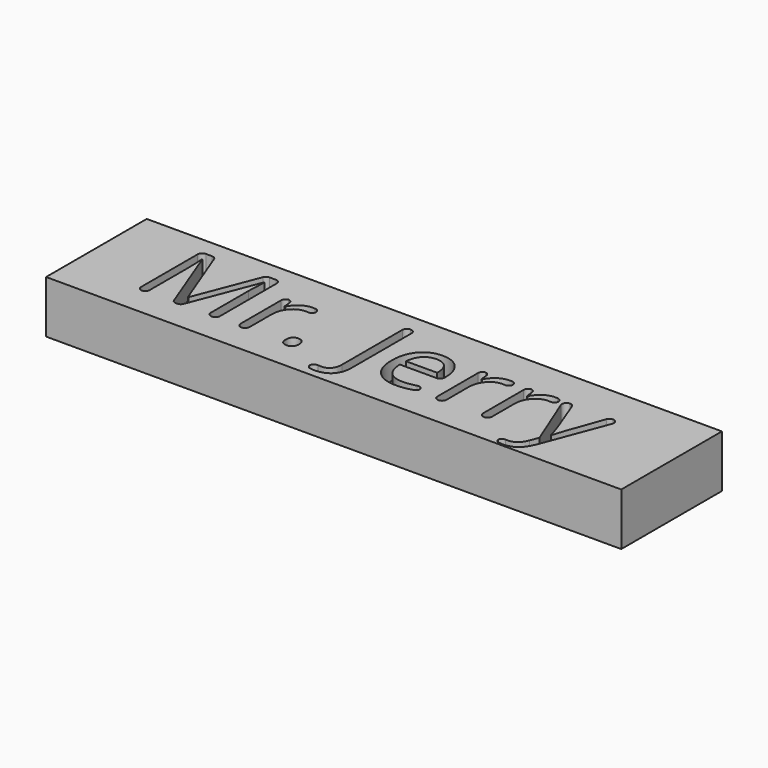
from build123d import *

# Parameters (mm, degrees)
F0_W         = 203.2
F0_H         = 44.45
F1_DEPTH     = 18.542
F2_TEXT_SIZE = 39.4664945685
F3_DEPTH     = 6.35
F4_T1_DEPTH  = 10.31875
F4_T3_DEPTH  = 9.0775000668
F4_T5_DEPTH  = 9.0694093583
F4_T7_DEPTH  = 9.9608913687
F4_T9_DEPTH  = 10.7046893029
F4_T11_DEPTH = 9.0805717525
F4_T13_DEPTH = 9.0709488545
F4_T15_DEPTH = 10.3720428243
F4_T17_DEPTH = 11.118182573
F4_T19_DEPTH = 9.8149761464
F4_T21_DEPTH = 9.1515288397
F4_T23_DEPTH = 11.9961106327
F4_T25_DEPTH = 9.0772375282
F4_T27_DEPTH = 9.1351619344
F4_T29_DEPTH = 12.2189306732
F4_T31_DEPTH = 12.0899797084
F4_T33_DEPTH = 10.8409697131
F4_T35_DEPTH = 9.9077155537


# Not quite as in the source:
# - a fillet or chamfer that OpenCascade refuses, or shapes differently, is made with other operations: its cross-section is extruded or revolved along the edge and cut away or added
# - Text() gives the source's letters only with a copy of the font that has no kerning and outlines rounded to 1/6400 em; it was checked with that copy


with BuildPart() as f1:
    # F0 (on Top) → F1 (new body)
    with BuildSketch(Plane.XY):
        with Locations((101.6, 22.225)):
            Rectangle(F0_W, F0_H)
    extrude(amount=F1_DEPTH)

    # F2 (on face) → F3 (cut)
    with BuildSketch(Plane.XY.offset(18.542)):
        with Locations((20.3022701502, 10.1437785078)):
            Text('Mr. Jerry', F2_TEXT_SIZE, font='Open Sans', text_align=(TextAlign.LEFT, TextAlign.BOTTOM))
    extrude(amount=-F3_DEPTH, mode=Mode.SUBTRACT)

    # F4: fillet of radius 1.5875 on 41 edges, made by hand

    # F4_s2 → F4_t1 (join)
    with BuildSketch(Plane.XY.offset(8.22325)):
        with BuildLine():
            ThreePointArc((25.7624199297, 38.3191556458), (24.6398879146, 37.8541876609), (24.1749199297, 36.7316556458))
            Line((24.1749199297, 36.7316556458), (24.1431699297, 36.7316556458))
            Line((24.1431699297, 36.7316556458), (24.1431699297, 38.3509056458))
            Line((24.1431699297, 38.3509056458), (25.7624199297, 38.3509056458))
            Line((25.7624199297, 38.3509056458), (25.7624199297, 38.3191556458))
        make_face()
        with BuildLine():
            ThreePointArc((52.0789649176, 36.7316556458), (51.6139969327, 37.8541876609), (50.4914649176, 38.3191556458))
            Line((50.4914649176, 38.3191556458), (50.4914649176, 38.3509056458))
            Line((50.4914649176, 38.3509056458), (52.1107149176, 38.3509056458))
            Line((52.1107149176, 38.3509056458), (52.1107149176, 36.7316556458))
            Line((52.1107149176, 36.7316556458), (52.0789649176, 36.7316556458))
        make_face()
        with BuildLine():
            ThreePointArc((60.9122666547, 31.2645197417), (59.7897346396, 30.7995517568), (59.3247666547, 29.6770197417))
            Line((59.3247666547, 29.6770197417), (59.2930166547, 29.6770197417))
            Line((59.2930166547, 29.6770197417), (59.2930166547, 31.2962697417))
            Line((59.2930166547, 31.2962697417), (60.9122666547, 31.2962697417))
            Line((60.9122666547, 31.2962697417), (60.9122666547, 31.2645197417))
        make_face()
        with BuildLine():
            ThreePointArc((25.6152400599, 10.1437785078), (26.737772075, 10.6087464926), (27.2027400599, 11.7312785078))
            Line((27.2027400599, 11.7312785078), (27.2344900599, 11.7312785078))
            Line((27.2344900599, 11.7312785078), (27.2344900599, 10.1120285078))
            Line((27.2344900599, 10.1120285078), (25.6152400599, 10.1120285078))
            Line((25.6152400599, 10.1120285078), (25.6152400599, 10.1437785078))
        make_face()
        with BuildLine():
            ThreePointArc((24.1749199297, 11.7312785078), (24.6398879146, 10.6087464926), (25.7624199297, 10.1437785078))
            Line((25.7624199297, 10.1437785078), (25.7624199297, 10.1120285078))
            Line((25.7624199297, 10.1120285078), (24.1431699297, 10.1120285078))
            Line((24.1431699297, 10.1120285078), (24.1431699297, 11.7312785078))
            Line((24.1431699297, 11.7312785078), (24.1749199297, 11.7312785078))
        make_face()
        with BuildLine():
            ThreePointArc((48.8044791963, 11.7312785078), (49.2694471812, 10.6087464926), (50.3919791963, 10.1437785078))
            Line((50.3919791963, 10.1437785078), (50.3919791963, 10.1120285078))
            Line((50.3919791963, 10.1120285078), (48.7727291963, 10.1120285078))
            Line((48.7727291963, 10.1120285078), (48.7727291963, 11.7312785078))
            Line((48.7727291963, 11.7312785078), (48.8044791963, 11.7312785078))
        make_face()
        with BuildLine():
            ThreePointArc((60.9377526987, 10.1437785078), (62.0602847138, 10.6087464926), (62.5252526987, 11.7312785078))
            Line((62.5252526987, 11.7312785078), (62.5570026987, 11.7312785078))
            Line((62.5570026987, 11.7312785078), (62.5570026987, 10.1120285078))
            Line((62.5570026987, 10.1120285078), (60.9377526987, 10.1120285078))
            Line((60.9377526987, 10.1120285078), (60.9377526987, 10.1437785078))
        make_face()
        with BuildLine():
            ThreePointArc((50.4914649176, 10.1437785078), (51.6139969327, 10.6087464926), (52.0789649176, 11.7312785078))
            Line((52.0789649176, 11.7312785078), (52.1107149176, 11.7312785078))
            Line((52.1107149176, 11.7312785078), (52.1107149176, 10.1120285078))
            Line((52.1107149176, 10.1120285078), (50.4914649176, 10.1120285078))
            Line((50.4914649176, 10.1120285078), (50.4914649176, 10.1437785078))
        make_face()
        with BuildLine():
            ThreePointArc((59.3247666547, 11.7312785078), (59.7897346396, 10.6087464926), (60.9122666547, 10.1437785078))
            Line((60.9122666547, 10.1437785078), (60.9122666547, 10.1120285078))
            Line((60.9122666547, 10.1120285078), (59.2930166547, 10.1120285078))
            Line((59.2930166547, 10.1120285078), (59.2930166547, 11.7312785078))
            Line((59.2930166547, 11.7312785078), (59.3247666547, 11.7312785078))
        make_face()
        with BuildLine():
            ThreePointArc((98.0539380275, 38.3191556458), (96.9314060124, 37.8541876609), (96.4664380275, 36.7316556458))
            Line((96.4664380275, 36.7316556458), (96.4346880275, 36.7316556458))
            Line((96.4346880275, 36.7316556458), (96.4346880275, 38.3509056458))
            Line((96.4346880275, 38.3509056458), (98.0539380275, 38.3509056458))
            Line((98.0539380275, 38.3509056458), (98.0539380275, 38.3191556458))
        make_face()
        with BuildLine():
            ThreePointArc((99.7409237488, 36.7316556458), (99.2759557639, 37.8541876609), (98.1534237488, 38.3191556458))
            Line((98.1534237488, 38.3191556458), (98.1534237488, 38.3509056458))
            Line((98.1534237488, 38.3509056458), (99.7726737488, 38.3509056458))
            Line((99.7726737488, 38.3509056458), (99.7726737488, 36.7316556458))
            Line((99.7726737488, 36.7316556458), (99.7409237488, 36.7316556458))
        make_face()
        with BuildLine():
            ThreePointArc((121.8333204898, 20.1275683056), (122.955852505, 20.5925362905), (123.4208204898, 21.7150683056))
            Line((123.4208204898, 21.7150683056), (123.4525704898, 21.7150683056))
            Line((123.4525704898, 21.7150683056), (123.4525704898, 20.0958183056))
            Line((123.4525704898, 20.0958183056), (121.8333204898, 20.0958183056))
            Line((121.8333204898, 20.0958183056), (121.8333204898, 20.1275683056))
        make_face()
        with BuildLine():
            ThreePointArc((130.4657966919, 31.2645197417), (129.3432646767, 30.7995517568), (128.8782966919, 29.6770197417))
            Line((128.8782966919, 29.6770197417), (128.8465466919, 29.6770197417))
            Line((128.8465466919, 29.6770197417), (128.8465466919, 31.2962697417))
            Line((128.8465466919, 31.2962697417), (130.4657966919, 31.2962697417))
            Line((130.4657966919, 31.2962697417), (130.4657966919, 31.2645197417))
        make_face()
        with BuildLine():
            ThreePointArc((128.8782966919, 11.7312785078), (129.3432646767, 10.6087464926), (130.4657966919, 10.1437785078))
            Line((130.4657966919, 10.1437785078), (130.4657966919, 10.1120285078))
            Line((130.4657966919, 10.1120285078), (128.8465466919, 10.1120285078))
            Line((128.8465466919, 10.1120285078), (128.8465466919, 11.7312785078))
            Line((128.8465466919, 11.7312785078), (128.8782966919, 11.7312785078))
        make_face()
        with BuildLine():
            ThreePointArc((130.4912827358, 10.1437785078), (131.6138147509, 10.6087464926), (132.0787827358, 11.7312785078))
            Line((132.0787827358, 11.7312785078), (132.1105327358, 11.7312785078))
            Line((132.1105327358, 11.7312785078), (132.1105327358, 10.1120285078))
            Line((132.1105327358, 10.1120285078), (130.4912827358, 10.1120285078))
            Line((130.4912827358, 10.1120285078), (130.4912827358, 10.1437785078))
        make_face()
        with BuildLine():
            ThreePointArc((146.5792264274, 31.2645197417), (145.4566944123, 30.7995517568), (144.9917264274, 29.6770197417))
            Line((144.9917264274, 29.6770197417), (144.9599764274, 29.6770197417))
            Line((144.9599764274, 29.6770197417), (144.9599764274, 31.2962697417))
            Line((144.9599764274, 31.2962697417), (146.5792264274, 31.2962697417))
            Line((146.5792264274, 31.2962697417), (146.5792264274, 31.2645197417))
        make_face()
        with BuildLine():
            ThreePointArc((144.9917264274, 11.7312785078), (145.4566944123, 10.6087464926), (146.5792264274, 10.1437785078))
            Line((146.5792264274, 10.1437785078), (146.5792264274, 10.1120285078))
            Line((146.5792264274, 10.1120285078), (144.9599764274, 10.1120285078))
            Line((144.9599764274, 10.1120285078), (144.9599764274, 11.7312785078))
            Line((144.9599764274, 11.7312785078), (144.9917264274, 11.7312785078))
        make_face()
        with BuildLine():
            ThreePointArc((146.6047124713, 10.1437785078), (147.7272444864, 10.6087464926), (148.1922124713, 11.7312785078))
            Line((148.1922124713, 11.7312785078), (148.2239624713, 11.7312785078))
            Line((148.2239624713, 11.7312785078), (148.2239624713, 10.1120285078))
            Line((148.2239624713, 10.1120285078), (146.6047124713, 10.1120285078))
            Line((146.6047124713, 10.1120285078), (146.6047124713, 10.1437785078))
        make_face()
    extrude(amount=F4_T1_DEPTH)

    # F4_s4 → F4_t3 (join)
    with BuildSketch(Plane.XY.offset(9.4644999332)):
        with BuildLine():
            ThreePointArc((29.4992621736, 37.3006389465), (28.9163688827, 38.0399784729), (28.0172317241, 38.3191556458))
            Line((28.0172317241, 38.3191556458), (28.0172317241, 38.3509056458))
            Line((28.0172317241, 38.3509056458), (29.1300517513, 38.3509056458))
            Line((29.1300517513, 38.3509056458), (29.5289027826, 37.3120186125))
            Line((29.5289027826, 37.3120186125), (29.4992621736, 37.3006389465))
        make_face()
    extrude(amount=F4_T3_DEPTH)

    # F4_s6 → F4_t5 (join)
    with BuildSketch(Plane.XY.offset(9.4725906417)):
        with BuildLine():
            ThreePointArc((48.2704166785, 38.3191556458), (47.3730936562, 38.0412233774), (46.7899690882, 37.3047448032))
            Line((46.7899690882, 37.3047448032), (46.7603601364, 37.3162065863))
            Line((46.7603601364, 37.3162065863), (47.1608976603, 38.3509056458))
            Line((47.1608976603, 38.3509056458), (48.2704166785, 38.3509056458))
            Line((48.2704166785, 38.3509056458), (48.2704166785, 38.3191556458))
        make_face()
    extrude(amount=F4_T5_DEPTH)

    # F4_s8 → F4_t7 (join)
    with BuildSketch(Plane.XY.offset(8.5811086313)):
        with BuildLine():
            ThreePointArc((62.100170343, 29.8265880456), (61.588075642, 30.8512420231), (60.5197319315, 31.2645197417))
            Line((60.5197319315, 31.2645197417), (60.5197319315, 31.2962697417))
            Line((60.5197319315, 31.2962697417), (61.99297561, 31.2962697417))
            Line((61.99297561, 31.2962697417), (62.1317791112, 29.8295794117))
            Line((62.1317791112, 29.8295794117), (62.100170343, 29.8265880456))
        make_face()
        with BuildLine():
            ThreePointArc((131.6537003801, 29.8265880456), (131.1416056791, 30.8512420231), (130.0732619686, 31.2645197417))
            Line((130.0732619686, 31.2645197417), (130.0732619686, 31.2962697417))
            Line((130.0732619686, 31.2962697417), (131.5465056471, 31.2962697417))
            Line((131.5465056471, 31.2962697417), (131.6853091483, 29.8295794117))
            Line((131.6853091483, 29.8295794117), (131.6537003801, 29.8265880456))
        make_face()
        with BuildLine():
            ThreePointArc((147.7671301156, 29.8265880456), (147.2550354147, 30.8512420231), (146.1866917042, 31.2645197417))
            Line((146.1866917042, 31.2645197417), (146.1866917042, 31.2962697417))
            Line((146.1866917042, 31.2962697417), (147.6599353826, 31.2962697417))
            Line((147.6599353826, 31.2962697417), (147.7987388839, 29.8295794117))
            Line((147.7987388839, 29.8295794117), (147.7671301156, 29.8265880456))
        make_face()
    extrude(amount=F4_T7_DEPTH)

    # F4_s10 → F4_t9 (join)
    with BuildSketch(Plane.XY.offset(7.8373106971)):
        with BuildLine():
            ThreePointArc((69.7567620656, 31.633185269), (70.9040374696, 31.0525772552), (71.2449954189, 29.8127812256))
            Line((71.2449954189, 29.8127812256), (71.2763955831, 29.8080809931))
            Line((71.2763955831, 29.8080809931), (71.5167804579, 31.4139855036))
            Line((71.5167804579, 31.4139855036), (71.4919038216, 31.4497583298))
            ThreePointArc((71.4919038216, 31.4497583298), (70.6289396634, 31.590880749), (69.7583975628, 31.6648931174))
            Line((69.7583975628, 31.6648931174), (69.7567620656, 31.633185269))
        make_face()
        with BuildLine():
            ThreePointArc((139.3102921027, 31.633185269), (140.4575675067, 31.0525772552), (140.798525456, 29.8127812256))
            Line((140.798525456, 29.8127812256), (140.8299256203, 29.8080809931))
            Line((140.8299256203, 29.8080809931), (141.070310495, 31.4139855036))
            Line((141.070310495, 31.4139855036), (141.0454338587, 31.4497583298))
            ThreePointArc((141.0454338587, 31.4497583298), (140.1824697005, 31.590880749), (139.3119275999, 31.6648931174))
            Line((139.3119275999, 31.6648931174), (139.3102921027, 31.633185269))
        make_face()
        with BuildLine():
            ThreePointArc((155.4237218383, 31.633185269), (156.5709972423, 31.0525772552), (156.9119551916, 29.8127812256))
            Line((156.9119551916, 29.8127812256), (156.9433553558, 29.8080809931))
            Line((156.9433553558, 29.8080809931), (157.1837402305, 31.4139855036))
            Line((157.1837402305, 31.4139855036), (157.1588635943, 31.4497583298))
            ThreePointArc((157.1588635943, 31.4497583298), (156.2958994361, 31.590880749), (155.4253573354, 31.6648931174))
            Line((155.4253573354, 31.6648931174), (155.4237218383, 31.633185269))
        make_face()
    extrude(amount=F4_T9_DEPTH)

    # F4_s12 → F4_t11 (join)
    with BuildSketch(Plane.XY.offset(9.4614282475)):
        with BuildLine():
            ThreePointArc((36.2534666318, 11.1638531198), (36.836269707, 10.4234283532), (37.7360942584, 10.1437785078))
            Line((37.7360942584, 10.1437785078), (37.7360942584, 10.1120285078))
            Line((37.7360942584, 10.1120285078), (36.6220209834, 10.1120285078))
            Line((36.6220209834, 10.1120285078), (36.2238140793, 11.1525046121))
            Line((36.2238140793, 11.1525046121), (36.2534666318, 11.1638531198))
        make_face()
    extrude(amount=F4_T11_DEPTH)

    # F4_s14 → F4_t13 (join)
    with BuildSketch(Plane.XY.offset(9.4710511455)):
        with BuildLine():
            ThreePointArc((38.1948078399, 10.1437785078), (39.092476454, 10.4219476446), (39.6755577251, 11.1589708741))
            Line((39.6755577251, 11.1589708741), (39.7051727228, 11.1475247214))
            Line((39.7051727228, 11.1475247214), (39.3049549725, 10.1120285078))
            Line((39.3049549725, 10.1120285078), (38.1948078399, 10.1120285078))
            Line((38.1948078399, 10.1120285078), (38.1948078399, 10.1437785078))
        make_face()
    extrude(amount=F4_T13_DEPTH)

    # F4_s16 → F4_t15 (join)
    with BuildSketch(Plane.XY.offset(8.1699571757)):
        with BuildLine():
            ThreePointArc((69.5517115576, 28.6989993236), (70.6845105226, 29.0258007119), (71.2795496167, 30.0436224639))
            Line((71.2795496167, 30.0436224639), (71.310949781, 30.0389222314))
            Line((71.310949781, 30.0389222314), (71.072782394, 28.4478317712))
            Line((71.072782394, 28.4478317712), (71.0345101701, 28.421534628))
            ThreePointArc((71.0345101701, 28.421534628), (70.2949645235, 28.5663493545), (69.5485549606, 28.6674066283))
            Line((69.5485549606, 28.6674066283), (69.5517115576, 28.6989993236))
        make_face()
        with BuildLine():
            ThreePointArc((139.1052415947, 28.6989993236), (140.2380405597, 29.0258007119), (140.8330796539, 30.0436224639))
            Line((140.8330796539, 30.0436224639), (140.8644798181, 30.0389222314))
            Line((140.8644798181, 30.0389222314), (140.6263124311, 28.4478317712))
            Line((140.6263124311, 28.4478317712), (140.5880402072, 28.421534628))
            ThreePointArc((140.5880402072, 28.421534628), (139.8484945606, 28.5663493545), (139.1020849978, 28.6674066283))
            Line((139.1020849978, 28.6674066283), (139.1052415947, 28.6989993236))
        make_face()
        with BuildLine():
            ThreePointArc((155.2186713302, 28.6989993236), (156.3514702952, 29.0258007119), (156.9465093894, 30.0436224639))
            Line((156.9465093894, 30.0436224639), (156.9779095536, 30.0389222314))
            Line((156.9779095536, 30.0389222314), (156.7397421667, 28.4478317712))
            Line((156.7397421667, 28.4478317712), (156.7014699427, 28.421534628))
            ThreePointArc((156.7014699427, 28.421534628), (155.9619242962, 28.5663493545), (155.2155147333, 28.6674066283))
            Line((155.2155147333, 28.6674066283), (155.2186713302, 28.6989993236))
        make_face()
    extrude(amount=F4_T15_DEPTH)

    # F4_s18 → F4_t17 (join)
    with BuildSketch(Plane.XY.offset(7.423817427)):
        with BuildLine():
            ThreePointArc((91.4663418723, 5.7090701886), (90.2426909962, 5.3068306582), (89.7201341122, 4.1295233875))
            Line((89.7201341122, 4.1295233875), (89.6883841122, 4.1295233875))
            Line((89.6883841122, 4.1295233875), (89.6883841122, 6.0367964167))
            Line((89.6883841122, 6.0367964167), (89.7286744232, 6.06737624))
            ThreePointArc((89.7286744232, 6.06737624), (90.5920257466, 5.8664611637), (91.4695160275, 5.7406611247))
            Line((91.4695160275, 5.7406611247), (91.4663418723, 5.7090701886))
        make_face()
    extrude(amount=F4_T17_DEPTH)

    # F4_s20 → F4_t19 (join)
    with BuildSketch(Plane.XY.offset(8.7270238536)):
        with BuildLine():
            ThreePointArc((91.045753848, 2.8387077239), (90.0960460697, 3.3786851317), (89.7201341122, 4.4044583353))
            Line((89.7201341122, 4.4044583353), (89.6883841122, 4.4044583353))
            Line((89.6883841122, 4.4044583353), (89.6883841122, 3.2433085981))
            Line((89.6883841122, 3.2433085981), (89.7060024142, 3.2148769676))
            ThreePointArc((89.7060024142, 3.2148769676), (90.3595642085, 2.961950272), (91.0405162427, 2.8073927116))
            Line((91.0405162427, 2.8073927116), (91.045753848, 2.8387077239))
        make_face()
    extrude(amount=F4_T19_DEPTH)

    # F4_s22 → F4_t21 (join)
    with BuildSketch(Plane.XY.offset(9.3904711603)):
        with BuildLine():
            ThreePointArc((121.4732914072, 10.7095207713), (122.2282990979, 11.2909791592), (122.5143244427, 12.2000005956))
            Line((122.5143244427, 12.2000005956), (122.5460744427, 12.2000005956))
            Line((122.5460744427, 12.2000005956), (122.5460744427, 11.1242742322))
            Line((122.5460744427, 11.1242742322), (122.5268441843, 11.0950968682))
            ThreePointArc((122.5268441843, 11.0950968682), (122.0083657121, 10.8803975141), (121.4842207465, 10.6797111748))
            Line((121.4842207465, 10.6797111748), (121.4732914072, 10.7095207713))
        make_face()
    extrude(amount=F4_T21_DEPTH)

    # F4_s24 → F4_t23 (join)
    with BuildSketch(Plane.XY.offset(6.5458893673)):
        with BuildLine():
            ThreePointArc((122.5143244427, 11.7209841956), (121.8772284967, 12.992553456), (120.4772997067, 13.2435096508))
            Line((120.4772997067, 13.2435096508), (120.468309212, 13.2739601599))
            ThreePointArc((120.468309212, 13.2739601599), (121.4958069444, 13.6114832276), (122.5018370805, 14.0086196851))
            Line((122.5018370805, 14.0086196851), (122.5460744427, 13.9794284486))
            Line((122.5460744427, 13.9794284486), (122.5460744427, 11.7209841956))
            Line((122.5460744427, 11.7209841956), (122.5143244427, 11.7209841956))
        make_face()
    extrude(amount=F4_T23_DEPTH)

    # F4_s26 → F4_t25 (join)
    with BuildSketch(Plane.XY.offset(9.4647624718)):
        with BuildLine():
            ThreePointArc((161.5764067813, 30.2461362211), (160.993505841, 30.9853829675), (160.0944274688, 31.2645197417))
            Line((160.0944274688, 31.2645197417), (160.0944274688, 31.2962697417))
            Line((160.0944274688, 31.2962697417), (161.2071403802, 31.2962697417))
            Line((161.2071403802, 31.2962697417), (161.6060463675, 30.2575185507))
            Line((161.6060463675, 30.2575185507), (161.5764067813, 30.2461362211))
        make_face()
    extrude(amount=F4_T25_DEPTH)

    # F4_s28 → F4_t27 (join)
    with BuildSketch(Plane.XY.offset(9.4068380656)):
        with BuildLine():
            ThreePointArc((175.2491739069, 31.2645197417), (174.3372785859, 30.9764823896), (173.7562933922, 30.2168938185))
            Line((173.7562933922, 30.2168938185), (173.7264357819, 30.2276913))
            ThreePointArc((173.7264357819, 30.2276913), (173.9158977523, 30.7515164316), (174.105410497, 31.27532302))
            Line((174.105410497, 31.27532302), (174.1352660103, 31.2962697417))
            Line((174.1352660103, 31.2962697417), (175.2491739069, 31.2962697417))
            Line((175.2491739069, 31.2962697417), (175.2491739069, 31.2645197417))
        make_face()
    extrude(amount=F4_T27_DEPTH)

    # F4_s30 → F4_t29 (join)
    with BuildSketch(Plane.XY.offset(6.3230693268)):
        with BuildLine():
            ThreePointArc((160.0980763939, 31.2645197417), (158.7830299739, 30.5662942569), (158.6247696001, 29.0858147507))
            Line((158.6247696001, 29.0858147507), (158.5953034642, 29.0739906508))
            Line((158.5953034642, 29.0739906508), (157.7035526792, 31.2962697417))
            Line((157.7035526792, 31.2962697417), (160.0980763939, 31.2962697417))
            Line((160.0980763939, 31.2962697417), (160.0980763939, 31.2645197417))
        make_face()
    extrude(amount=F4_T29_DEPTH)

    # F4_s32 → F4_t31 (join)
    with BuildSketch(Plane.XY.offset(6.4520202916)):
        with BuildLine():
            ThreePointArc((176.753155592, 29.1164407183), (176.5736967738, 30.5798588886), (175.2679258426, 31.2645197417))
            Line((175.2679258426, 31.2645197417), (175.2679258426, 31.2962697417))
            Line((175.2679258426, 31.2962697417), (177.6098375636, 31.2962697417))
            Line((177.6098375636, 31.2962697417), (176.782860187, 29.1052291378))
            Line((176.782860187, 29.1052291378), (176.753155592, 29.1164407183))
        make_face()
    extrude(amount=F4_T31_DEPTH)

    # F4_s34 → F4_t33 (join)
    with BuildSketch(Plane.XY.offset(7.7010302869)):
        with BuildLine():
            ThreePointArc((159.6895796752, 3.3407233721), (158.5155424524, 2.9058053185), (158.0218362748, 1.7552527017))
            Line((158.0218362748, 1.7552527017), (157.9900862748, 1.7552527017))
            Line((157.9900862748, 1.7552527017), (157.9900862748, 3.5516405869))
            Line((157.9900862748, 3.5516405869), (158.0285134701, 3.5826805218))
            ThreePointArc((158.0285134701, 3.5826805218), (158.8554589217, 3.4441687406), (159.6911845432, 3.3724327855))
            Line((159.6911845432, 3.3724327855), (159.6895796752, 3.3407233721))
        make_face()
    extrude(amount=F4_T33_DEPTH)

    # F4_s36 → F4_t35 (join)
    with BuildSketch(Plane.XY.offset(8.6342844463)):
        with BuildLine():
            ThreePointArc((158.0218362748, 2.3232382873), (158.422928447, 1.268443181), (159.4235278858, 0.7466497257))
            Line((159.4235278858, 0.7466497257), (159.419811718, 0.7151179545))
            ThreePointArc((159.419811718, 0.7151179545), (158.7137383118, 0.8185934917), (158.0146090424, 0.9615685855))
            Line((158.0146090424, 0.9615685855), (157.9900862748, 0.9924850797))
            Line((157.9900862748, 0.9924850797), (157.9900862748, 2.3232382873))
            Line((157.9900862748, 2.3232382873), (158.0218362748, 2.3232382873))
        make_face()
    extrude(amount=F4_T35_DEPTH)


solid = f1.part
